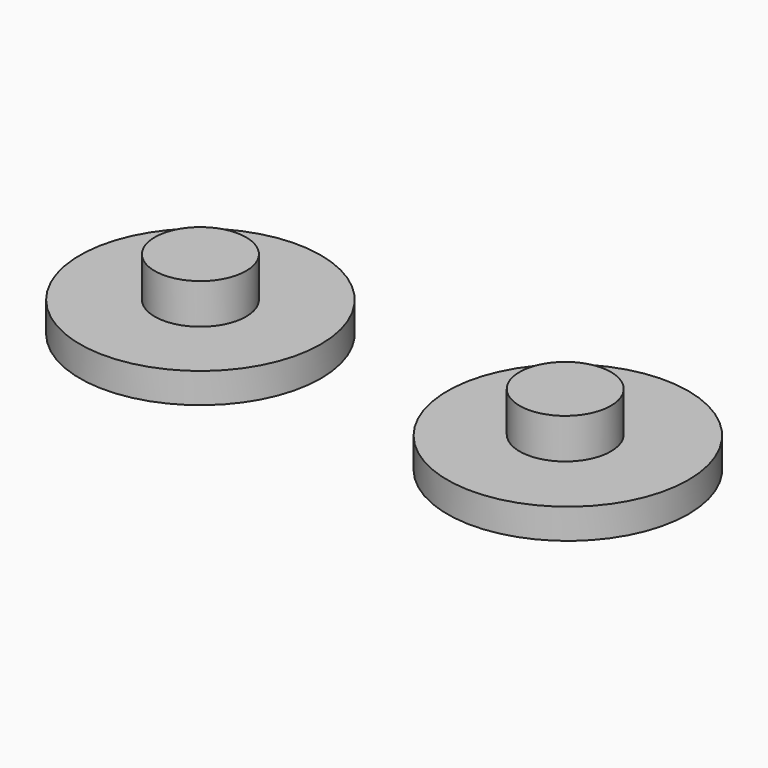
from build123d import *

# Parameters (mm, degrees)
F0_R     = 6
F1_DEPTH = 1.5
F2_R     = 2.275
F3_DEPTH = 3.5


with BuildPart() as f1:
    # F0 (on Top) → F1 (new body)
    with BuildSketch(Plane.XY):
        Circle(F0_R)
    extrude(amount=F1_DEPTH)

    # F2 (on Top) → F3 (join)
    with BuildSketch(Plane.XY):
        Circle(F2_R)
    extrude(amount=F3_DEPTH)


with BuildPart() as f1b:
    # F0 (on Top) → F1, piece 2 (new body)
    with BuildSketch(Plane.XY):
        with Locations((18.2954519987, 0)):
            Circle(F0_R)
    extrude(amount=F1_DEPTH)


with BuildPart() as f3:
    # F2 (on Top) → F3, piece 2 (new body)
    with BuildSketch(Plane.XY):
        with Locations((18.1653685868, 0)):
            Circle(F2_R)
    extrude(amount=F3_DEPTH)


solid = Compound([f1.part, f1b.part, f3.part])
